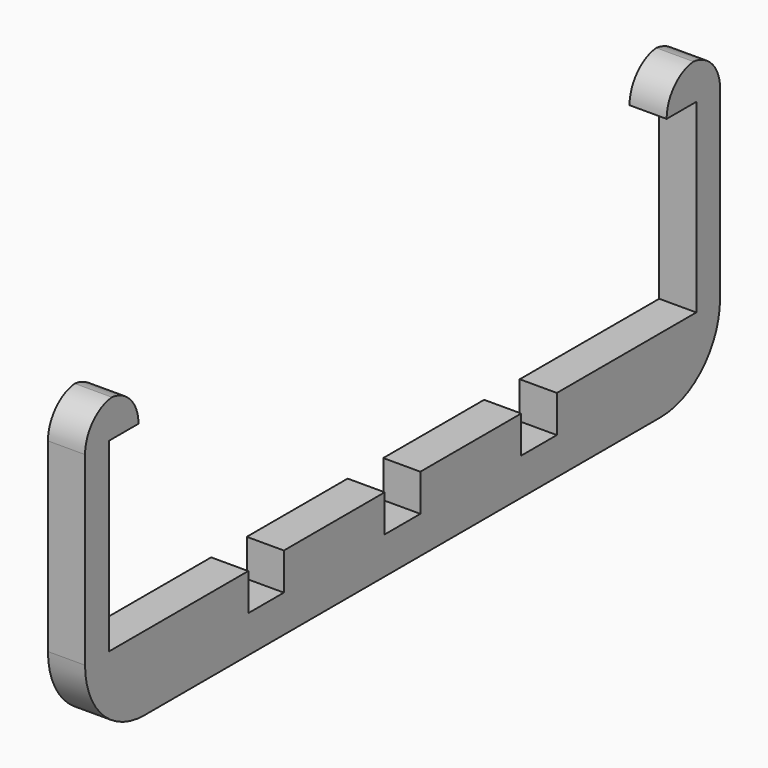
from build123d import *

# Parameters (mm, degrees)
F0_W         = 5
F0_H         = 107
F1_DEPTH     = 10
F3_W         = 5
F3_H         = 6
F4_DEPTH     = 5
F5_DEPTH     = 5
F6_R         = 9.99999
F2_W         = 5
F2_H         = 4
F7_DEPTH     = 30
F8_DEPTH     = 30
F9_W         = 5
F9_H         = 5
F10_DEPTH    = 5
F11_W        = 5
F11_H        = 5
F12_DEPTH    = 5
F13_T1_DEPTH = 30
F14_W        = 5
F14_H        = 6
F15_DEPTH    = 5


# Not quite as in the source:
# - a fillet or chamfer that OpenCascade refuses, or shapes differently, is made with other operations: its cross-section is extruded or revolved along the edge and cut away or added
# - a fillet or chamfer is up to 0.001 mm smaller than in the source, because OpenCascade refuses the exact size
# - a feature names something its author has since deleted; it is built from what else it names


with BuildPart() as f1:
    # F0 (on Top) → F1 (new body)
    with BuildSketch(Plane.XY):
        Rectangle(F0_W, F0_H)
    extrude(amount=F1_DEPTH)

    # F3 (on face) → F4 (cut)
    with BuildSketch(Plane.XY.offset(10)):
        with Locations((0, 23)):
            Rectangle(F3_W, F3_H)
    extrude(amount=-F4_DEPTH, mode=Mode.SUBTRACT)

    # F3 (on face) → F5 (cut)
    with BuildSketch(Plane.XY.offset(10)):
        with Locations((0, 23)):
            Rectangle(F3_W, F3_H)
        with Locations((0, -23)):
            Rectangle(F3_W, F3_H)
    extrude(amount=-F5_DEPTH, mode=Mode.SUBTRACT)

    # F6 (radius 10 in the source; OpenCascade refuses exactly that, so slightly less here)
    f6_edges = [f1.edges().sort_by_distance(p)[0] for p in [
        (0, -53.5, 0),
        (0, 53.5, 0),
    ]]
    fillet(f6_edges, radius=F6_R)

    # F2 (on face) → F7 (join)
    with BuildSketch(Plane.XY.offset(10)):
        with Locations((0, 51.5)):
            Rectangle(F2_W, F2_H)
    extrude(amount=F7_DEPTH)

    # F2 (on face) → F8 (join)
    with BuildSketch(Plane.XY.offset(10)):
        with Locations((0, 51.5)):
            Rectangle(F2_W, F2_H)
        with Locations((0, -51.5)):
            Rectangle(F2_W, F2_H)
    extrude(amount=F8_DEPTH)

    # F9 (on face) → F10 (join)
    with BuildSketch(Plane(origin=(0, -49.5, 0), x_dir=(-1, 0, 0), z_dir=(0, 1, 0))):
        with Locations((0, 37.5)):
            Rectangle(F9_W, F9_H)
    extrude(amount=F10_DEPTH)

    # F11 (on face) → F12 (join)
    with BuildSketch(Plane.XZ.offset(-49.5)):
        with Locations((0, 37.5)):
            Rectangle(F11_W, F11_H)
    extrude(amount=F12_DEPTH)

    # F13: fillet of radius 5 on 4 edges, made by hand

    # F13_s2 → F13_t1 (cut)
    with BuildSketch(Plane.YZ.offset(-15)):
        with BuildLine():
            ThreePointArc((-48.5, 40), (-52.0355339059, 38.5355339059), (-53.5, 35))
            Line((-53.5, 35), (-53.5, 40))
            Line((-53.5, 40), (-48.5, 40))
        make_face()
        with BuildLine():
            ThreePointArc((53.5, 35), (52.0355339059, 38.5355339059), (48.5, 40))
            Line((48.5, 40), (53.5, 40))
            Line((53.5, 40), (53.5, 35))
        make_face()
        with BuildLine():
            ThreePointArc((49.5, 40), (45.9644660941, 38.5355339059), (44.5, 35))
            Line((44.5, 35), (44.5, 40))
            Line((44.5, 40), (49.5, 40))
        make_face()
        with BuildLine():
            ThreePointArc((-44.5, 35), (-45.9644660941, 38.5355339059), (-49.5, 40))
            Line((-49.5, 40), (-44.5, 40))
            Line((-44.5, 40), (-44.5, 35))
        make_face()
    extrude(amount=F13_T1_DEPTH, mode=Mode.SUBTRACT)

    # F14 (on face) → F15 (cut)
    with BuildSketch(Plane.XY.offset(10)):
        Rectangle(F14_W, F14_H)
    extrude(amount=-F15_DEPTH, mode=Mode.SUBTRACT)


solid = f1.part
